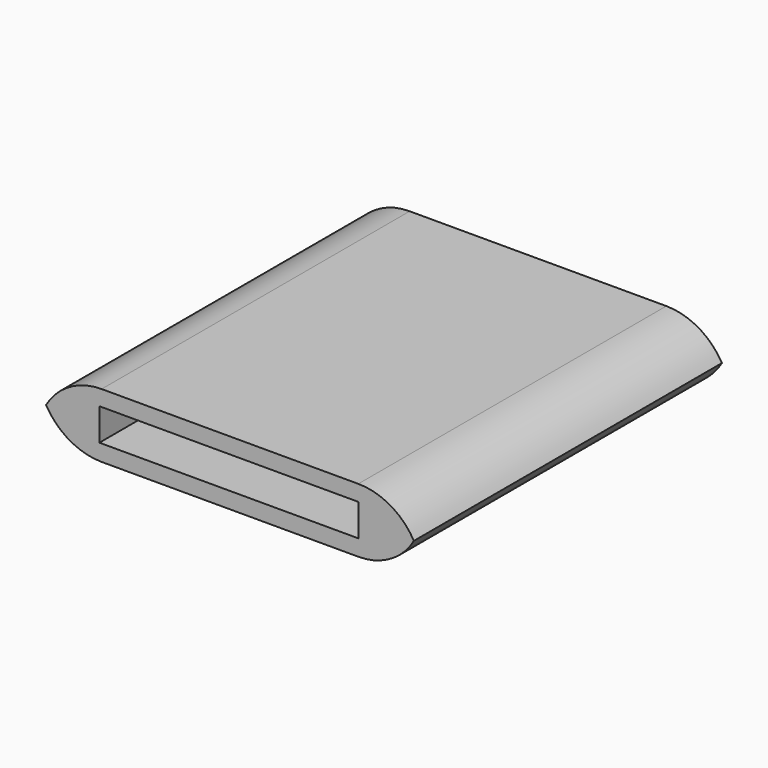
from build123d import *

# Parameters (mm, degrees)
F0_W        = 7.62
F0_H        = 7.62
F1_DEPTH    = 1.27
F2_T1_DEPTH = 13.97
F3_W        = 5.1244873625
F3_H        = 0.6355810037
F4_DEPTH    = 7.62


# Not quite as in the source:
# - a fillet or chamfer that OpenCascade refuses, or shapes differently, is made with other operations: its cross-section is extruded or revolved along the edge and cut away or added


with BuildPart() as f1:
    # F0 (on Top) → F1 (new body)
    with BuildSketch(Plane.XY):
        with Locations((-34.8768493396, 33.171152453)):
            Rectangle(F0_W, F0_H)
    extrude(amount=F1_DEPTH)

    # F2: fillet of radius 1.27 on 4 edges, made by hand

    # F2_s2 → F2_t1 (cut)
    with BuildSketch(Plane.XZ.offset(-40.156152453)):
        with BuildLine():
            ThreePointArc((-38.6868493396, 0), (-38.3148749517, 0.8980256121), (-37.4168493396, 1.27))
            Line((-37.4168493396, 1.27), (-38.6868493396, 1.27))
            Line((-38.6868493396, 1.27), (-38.6868493396, 0))
        make_face()
        with BuildLine():
            ThreePointArc((-31.0668493396, 0), (-31.4388237275, 0.8980256121), (-32.3368493396, 1.27))
            Line((-32.3368493396, 1.27), (-31.0668493396, 1.27))
            Line((-31.0668493396, 1.27), (-31.0668493396, 0))
        make_face()
        with BuildLine():
            ThreePointArc((-38.6868493396, 1.27), (-38.3148749517, 0.3719743879), (-37.4168493396, 0))
            Line((-37.4168493396, 0), (-38.6868493396, 0))
            Line((-38.6868493396, 0), (-38.6868493396, 1.27))
        make_face()
        with BuildLine():
            ThreePointArc((-31.0668493396, 1.27), (-31.4388237275, 0.3719743879), (-32.3368493396, 0))
            Line((-32.3368493396, 0), (-31.0668493396, 0))
            Line((-31.0668493396, 0), (-31.0668493396, 1.27))
        make_face()
    extrude(amount=F2_T1_DEPTH, mode=Mode.SUBTRACT)

    # F3 (on face) → F4 (cut)
    with BuildSketch(Plane(origin=(0, 36.981152453, 0), x_dir=(-1, 0, 0), z_dir=(0, 1, 0))):
        with Locations((34.8990930209, 0.6385907036)):
            Rectangle(F3_W, F3_H)
    extrude(amount=-F4_DEPTH, mode=Mode.SUBTRACT)


solid = f1.part
